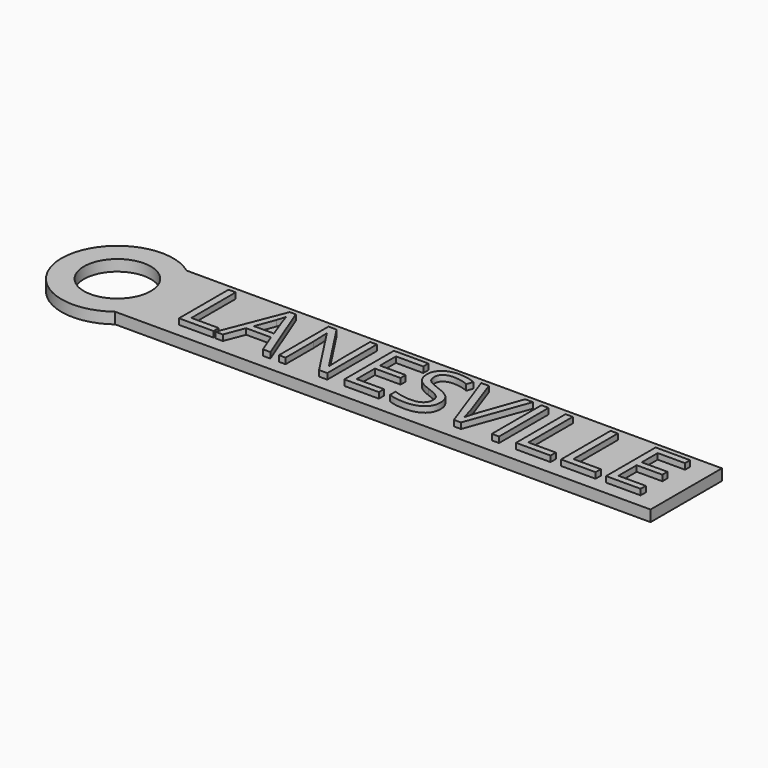
from build123d import *

# Parameters (mm, degrees)
F0_W         = 76.2
F0_H         = 12.7
F1_DEPTH     = 1.5875
F2_TEXT_SIZE = 12.3486225009
F3_DEPTH     = 0.8255
F4_R         = 7.9375
F4_R_2       = 4.7625
F5_DEPTH     = 1.5875


# Not quite as in the source:
# - Text() gives the source's letters only with a copy of the font that has no kerning and outlines rounded to 1/6400 em; it was checked with that copy


with BuildPart() as f1:
    # F0 (on Top) → F1 (new body)
    with BuildSketch(Plane.XY):
        Rectangle(F0_W, F0_H)
    extrude(amount=-F1_DEPTH)

    # F2 (on face) → F3 (join)
    with BuildSketch(Plane.XY):
        with Locations((-31.800495543, -4.3849541079)):
            Text('LANESVILLE', F2_TEXT_SIZE, font='Open Sans', text_align=(TextAlign.LEFT, TextAlign.BOTTOM))
    extrude(amount=F3_DEPTH)

    # F4 (on face) → F5 (join, through all)
    with BuildSketch(Plane.XY):
        with Locations((-42.8625, 0)):
            Circle(F4_R)
        with Locations((-42.8625, 0)):
            Circle(F4_R_2, mode=Mode.SUBTRACT)
    extrude(amount=-F5_DEPTH)


solid = f1.part
